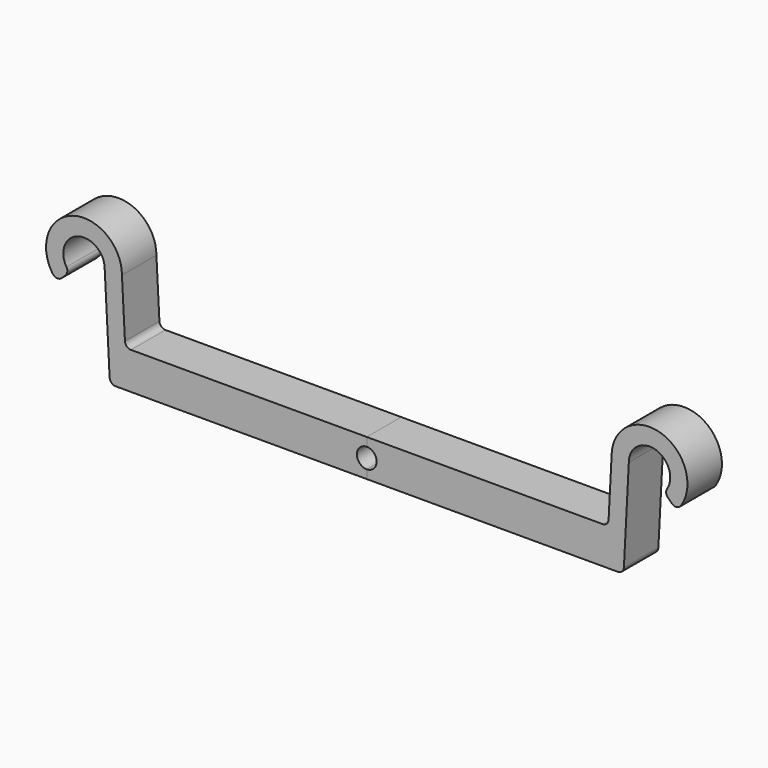
from build123d import *
from build123d import SkipClean  # not in build123d's __all__

# Parameters (mm, degrees)
F1_DEPTH = 5
F2_R     = 0.7


with BuildPart() as f1:
    # F0 (on Front) → F1 (new body)
    with BuildSketch(Plane.XZ):
        with BuildLine():
            Line((0, -1), (0, 0))
            Line((0, 0), (-28.0174232112, 0))
            Line((-28.0174232112, 0), (-28.4, 7.3))
            ThreePointArc((-28.4, 7.3), (-34.4838071024, 11.365069943), (-35.9112698372, 4.1887301628))
            Line((-35.9112698372, 4.1887301628), (-34.4970562748, 5.6029437252))
            ThreePointArc((-34.4970562748, 5.6029437252), (-33.7184402377, 9.517310878), (-30.4, 7.3))
            Line((-30.4, 7.3), (-29.7920697603, -4.3))
            Line((-29.7920697603, -4.3), (0, -4.3))
            Line((0, -4.3), (0, -3.3))
            ThreePointArc((0, -3.3), (-1.15, -2.15), (0, -1))
        make_face()
    extrude(amount=F1_DEPTH)

    # F2
    f2_edges = [f1.edges().sort_by_distance(p)[0] for p in [
        (-28.017423, -2.5, 0),
        (-29.79207, -2.5, -4.3),
        (-34.497056, -2.5, 5.602944),
        (-35.91127, -2.5, 4.18873),
    ]]
    fillet(f2_edges, radius=F2_R)

    # F3: F1 across plane


with BuildPart() as f1_1:
    add(f1.part, clean=False)
    with SkipClean():  # cleaning this boolean's faces spoils the solid; the shape is the same uncleaned
        add(f1.part.mirror(Plane.YZ), clean=False)


solid = f1_1.part
